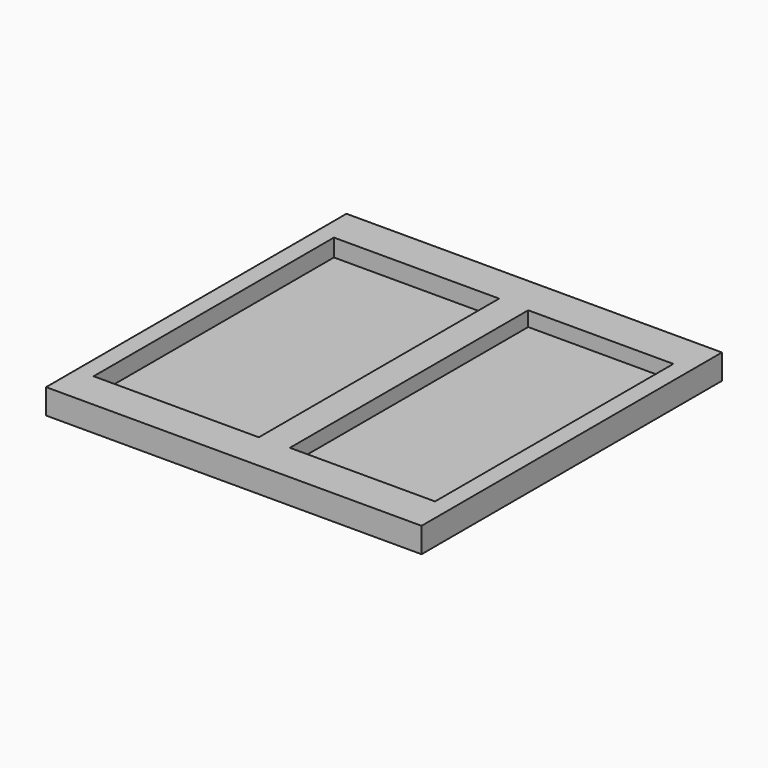
from build123d import *

# Parameters (mm, degrees)
F0_W     = 150
F0_H     = 150
F1_DEPTH = 10
F2_W     = 66
F2_H     = 120
F3_DEPTH = 7
F4_W     = 58
F4_H     = 119
F5_DEPTH = 5.9


# Not quite as in the source:
# - a feature names something its author has since deleted; it is built from what else it names


with BuildPart() as f1:
    # F0 (on Top) → F1 (new body)
    with BuildSketch(Plane.XY):
        Rectangle(F0_W, F0_H)
    extrude(amount=F1_DEPTH)

    # F2 (on face) → F3 (cut)
    with BuildSketch(Plane.XY.offset(10)):
        with Locations((-35, 0)):
            Rectangle(F2_W, F2_H)
    extrude(amount=-F3_DEPTH, mode=Mode.SUBTRACT)

    # F4 (on face) → F5 (cut)
    with BuildSketch(Plane.XY.offset(10)):
        with Locations((39, 0)):
            Rectangle(F4_W, F4_H)
    extrude(amount=-F5_DEPTH, mode=Mode.SUBTRACT)


solid = f1.part
